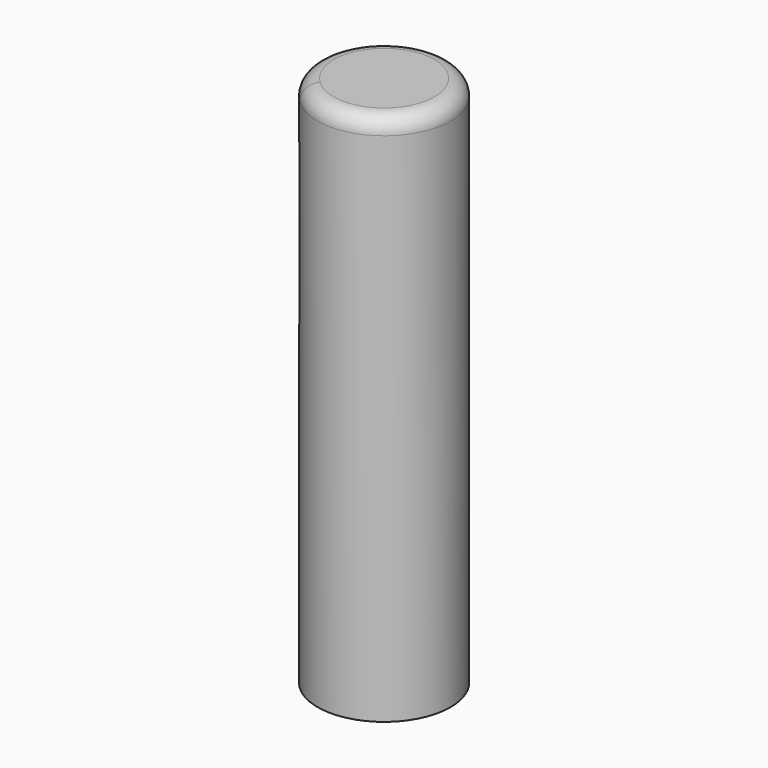
from build123d import *

# Parameters (mm, degrees)
F0_R         = 8.25
F0_R_2       = 6.25
F1_DEPTH     = 34
F2_R         = 8.25
F3_DEPTH     = 32
F5_DEPTH     = 28
F6_DEPTH     = 5
F7_T4_DEPTH  = 26
F7_S5_R      = 8.25
F7_T6_DEPTH  = 15
F7_T10_DEPTH = 26
F7_S11_R     = 8.25
F7_T12_DEPTH = 15
F8_R         = 2


# Not quite as in the source:
# - a fillet or chamfer that OpenCascade refuses, or shapes differently, is made with other operations: its cross-section is extruded or revolved along the edge and cut away or added


with BuildPart() as f1:
    # F0 (on Top) → F1 (new body)
    with BuildSketch(Plane.XY):
        Circle(F0_R)
        Circle(F0_R_2, mode=Mode.SUBTRACT)
    extrude(amount=F1_DEPTH)

    # F2 (on face) → F3 (join)
    with BuildSketch(Plane.XY.offset(34)):
        Circle(F2_R)
    extrude(amount=F3_DEPTH)

    # F4 (on face) → F5 (cut)
    with BuildSketch(Plane.XY.offset(66)):
        with BuildLine():
            Line((-5.6623758265, -6), (-5.6623758265, 6))
            ThreePointArc((-5.6623758265, 6), (-8.25, 0), (-5.6623758265, -6))
        make_face()
    extrude(amount=-F5_DEPTH, mode=Mode.SUBTRACT)

    # F4 (on face) → F6 (join)
    with BuildSketch(Plane.XY.offset(66)):
        with BuildLine():
            Line((-5.6623758265, -6), (-5.6623758265, 6))
            ThreePointArc((-5.6623758265, 6), (-8.25, 0), (-5.6623758265, -6))
        make_face()
    extrude(amount=-F6_DEPTH)

    # F7: fillet of radius 2.8 on 2 edges, made by hand


with BuildPart() as f7_tool2:
    # F7_s3 → F7_t4 (new body)
    with BuildSketch(Plane.XZ.offset(13)):
        with BuildLine():
            ThreePointArc((-8.4623758265, 61), (-6.4824768391, 60.1798989873), (-5.6623758265, 58.2))
            Line((-5.6623758265, 58.2), (-5.6623758265, 61))
            Line((-5.6623758265, 61), (-8.4623758265, 61))
        make_face()
    extrude(amount=-F7_T4_DEPTH)

    # F7_s5 → F7_t6 (intersect, symmetric)
    with BuildSketch(Plane.XY.offset(59.6)):
        Circle(F7_S5_R)
    extrude(amount=F7_T6_DEPTH, both=True, mode=Mode.INTERSECT)


with BuildPart() as f1_1:
    add(f1.part)

    # F7_t1: union F7_tool2
    add(f7_tool2.part)


with BuildPart() as f7_tool8:
    # F7_s9 → F7_t10 (new body)
    with BuildSketch(Plane.XZ.offset(13)):
        with BuildLine():
            ThreePointArc((-8.4623758265, 38), (-6.4824768391, 38.8201010127), (-5.6623758265, 40.8))
            Line((-5.6623758265, 40.8), (-5.6623758265, 38))
            Line((-5.6623758265, 38), (-8.4623758265, 38))
        make_face()
    extrude(amount=-F7_T10_DEPTH)

    # F7_s11 → F7_t12 (intersect, symmetric)
    with BuildSketch(Plane.XY.offset(39.4)):
        Circle(F7_S11_R)
    extrude(amount=F7_T12_DEPTH, both=True, mode=Mode.INTERSECT)


with BuildPart() as f1_2:
    add(f1_1.part)

    # F7_t7: union F7_tool8
    add(f7_tool8.part)

    # F8
    f8_edges = [f1_2.edges().sort_by_distance(p)[0] for p in [
        (-8.25, 0, 66),
    ]]
    fillet(f8_edges, radius=F8_R)


solid = f1_2.part
